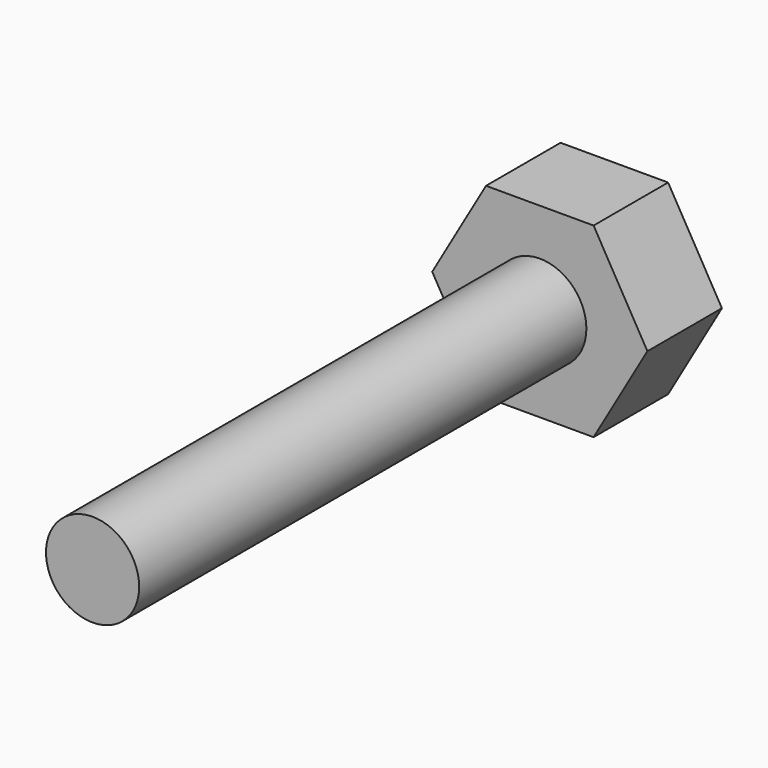
from build123d import *

# Parameters (mm, degrees)
F0_R     = 5
F1_DEPTH = 60
F2_R     = 5
F3_DEPTH = 10


with BuildPart() as f1:
    # F0 (on Front) → F1 (new body)
    with BuildSketch(Plane.XZ):
        Circle(F0_R)
    extrude(amount=F1_DEPTH)

    # F2 (on face) → F3 (join)
    with BuildSketch(Plane(origin=(0, 0, 0), x_dir=(-1, 0, 0), z_dir=(0, 1, 0))):
        Polygon((5.7735026919, -10), (11.5470053838, 0), (5.7735026919, 10), (-5.7735026919, 10), (-11.5470053838, 0), (-5.7735026919, -10), align=None)
        Circle(F2_R, mode=Mode.SUBTRACT)
        Circle(F2_R)
    extrude(amount=F3_DEPTH)


solid = f1.part
